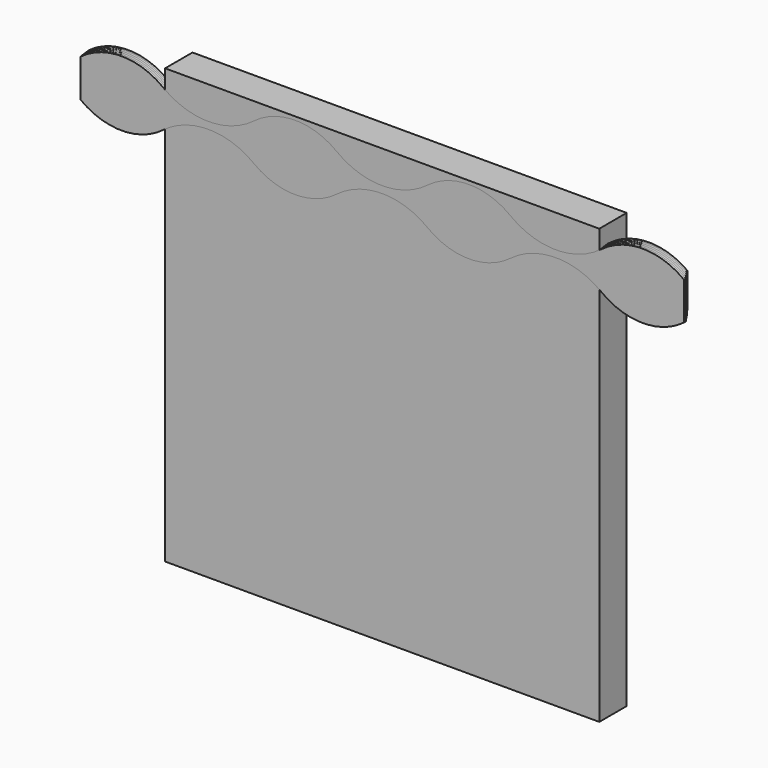
from build123d import *

# Parameters (mm, degrees)
F0_W      = 190
F0_H      = 190
F1_DEPTH  = 15
F3_DEPTH  = 1
F5_DEPTH  = 1
F7_DEPTH  = 1
F9_DEPTH  = 1
F11_DEPTH = 1


with BuildPart() as f1:
    # F0 (on Front) → F1 (new body)
    with BuildSketch(Plane.XZ):
        Rectangle(F0_W, F0_H)
    extrude(amount=-F1_DEPTH)


with BuildPart() as f3:
    # F2 (on face) → F3 (new body)
    with BuildSketch(Plane.XZ):
        with BuildLine():
            ThreePointArc((-56.0905668848, 87.3904664468), (-76, 80.6666666667), (-95.9094331152, 87.3904664468))
            ThreePointArc((-95.9094331152, 87.3904664468), (-114, 93.5), (-132.0905668848, 87.3904664468))
            Line((-132.0905668848, 87.3904664468), (-132.0905668848, 70.9428668865))
            ThreePointArc((-132.0905668848, 70.9428668865), (-114, 64.8333333333), (-95.9094331152, 70.9428668865))
            ThreePointArc((-95.9094331152, 70.9428668865), (-76, 77.6666666667), (-56.0905668848, 70.9428668865))
            ThreePointArc((-56.0905668848, 70.9428668865), (-38, 64.8333333333), (-19.9094331152, 70.9428668865))
            ThreePointArc((-19.9094331152, 70.9428668865), (0, 77.6666666667), (19.9094331152, 70.9428668865))
            ThreePointArc((19.9094331152, 70.9428668865), (38, 64.8333333333), (56.0905668848, 70.9428668865))
            ThreePointArc((56.0905668848, 70.9428668865), (76, 77.6666666667), (95.9094331152, 70.9428668865))
            ThreePointArc((95.9094331152, 70.9428668865), (114, 64.8333333333), (132.0905668848, 70.9428668865))
            Line((132.0905668848, 70.9428668865), (132.0905668848, 87.3904664468))
            ThreePointArc((132.0905668848, 87.3904664468), (114, 93.5), (95.9094331152, 87.3904664468))
            ThreePointArc((95.9094331152, 87.3904664468), (76, 80.6666666667), (56.0905668848, 87.3904664468))
            ThreePointArc((56.0905668848, 87.3904664468), (38, 93.5), (19.9094331152, 87.3904664468))
            ThreePointArc((19.9094331152, 87.3904664468), (0, 80.6666666667), (-19.9094331152, 87.3904664468))
            ThreePointArc((-19.9094331152, 87.3904664468), (-38, 93.5), (-56.0905668848, 87.3904664468))
        make_face()
    extrude(amount=-F3_DEPTH)

    # F4 (on face) → F5 (join)
    with BuildSketch(Plane(origin=(0, 1, 0), x_dir=(-1, 0, 0), z_dir=(0, 1, 0))):
        with BuildLine():
            ThreePointArc((-95.7913197263, 87.4518930814), (-113.6258792589, 93.4999070156), (-131.4905668729, 87.541474107))
            Line((-131.4905668729, 87.541474107), (-131.4905668729, 71.3918592502))
            ThreePointArc((-131.4905668729, 71.3918592502), (-113.6258792589, 65.4334263416), (-95.7913197263, 71.4814402758))
            ThreePointArc((-95.7913197263, 71.4814402758), (-75.6999999881, 78.2666666786), (-55.6086802499, 71.4814402758))
            ThreePointArc((-55.6086802499, 71.4814402758), (-37.6999999881, 65.4333333453), (-19.7913197263, 71.4814402758))
            ThreePointArc((-19.7913197263, 71.4814402758), (0.3000000119, 78.2666666786), (20.3913197501, 71.4814402758))
            ThreePointArc((20.3913197501, 71.4814402758), (38.3000000119, 65.4333333453), (56.2086802737, 71.4814402758))
            ThreePointArc((56.2086802737, 71.4814402758), (76.3000000119, 78.2666666786), (96.3913197501, 71.4814402758))
            ThreePointArc((96.3913197501, 71.4814402758), (114.2258792828, 65.4334263416), (132.0905668967, 71.3918592502))
            Line((132.0905668967, 71.3918592502), (132.0905668967, 87.541474107))
            ThreePointArc((132.0905668967, 87.541474107), (114.2258792828, 93.4999070156), (96.3913197501, 87.4518930814))
            ThreePointArc((96.3913197501, 87.4518930814), (76.3000000119, 80.6666666786), (56.2086802737, 87.4518930814))
            ThreePointArc((56.2086802737, 87.4518930814), (38.3000000119, 93.5000000119), (20.3913197501, 87.4518930814))
            ThreePointArc((20.3913197501, 87.4518930814), (0.3000000119, 80.6666666786), (-19.7913197263, 87.4518930814))
            ThreePointArc((-19.7913197263, 87.4518930814), (-37.6999999881, 93.5000000119), (-55.6086802499, 87.4518930814))
            ThreePointArc((-55.6086802499, 87.4518930814), (-75.6999999881, 80.6666666786), (-95.7913197263, 87.4518930814))
        make_face()
    extrude(amount=F5_DEPTH)

    # F6 (on face) → F7 (join)
    with BuildSketch(Plane(origin=(0, 2, 0), x_dir=(-1, 0, 0), z_dir=(0, 1, 0))):
        with BuildLine():
            ThreePointArc((56.3267936626, 87.513319716), (38.6000000238, 93.5000000238), (20.8732063851, 87.513319716))
            ThreePointArc((20.8732063851, 87.513319716), (0.6000000238, 80.6666666905), (-19.6732063374, 87.513319716))
            ThreePointArc((-19.6732063374, 87.513319716), (-37.3999999762, 93.5000000238), (-55.1267936149, 87.513319716))
            ThreePointArc((-55.1267936149, 87.513319716), (-75.3999999762, 80.6666666905), (-95.6732063374, 87.513319716))
            ThreePointArc((-95.6732063374, 87.513319716), (-113.2520443013, 93.4996256674), (-130.890566861, 87.6915343271))
            Line((-130.890566861, 87.6915343271), (-130.890566861, 71.8417990539))
            ThreePointArc((-130.890566861, 71.8417990539), (-113.2520443013, 66.0337077137), (-95.6732063374, 72.020013665))
            ThreePointArc((-95.6732063374, 72.020013665), (-75.3999999762, 78.8666666905), (-55.1267936149, 72.020013665))
            ThreePointArc((-55.1267936149, 72.020013665), (-37.3999999762, 66.0333333572), (-19.6732063374, 72.020013665))
            ThreePointArc((-19.6732063374, 72.020013665), (0.6000000238, 78.8666666905), (20.8732063851, 72.020013665))
            ThreePointArc((20.8732063851, 72.020013665), (38.6000000238, 66.0333333572), (56.3267936626, 72.020013665))
            ThreePointArc((56.3267936626, 72.020013665), (76.6000000238, 78.8666666905), (96.8732063851, 72.020013665))
            ThreePointArc((96.8732063851, 72.020013665), (114.452044349, 66.0337077137), (132.0905669087, 71.8417990539))
            Line((132.0905669087, 71.8417990539), (132.0905669087, 87.6915343271))
            ThreePointArc((132.0905669087, 87.6915343271), (114.452044349, 93.4996256674), (96.8732063851, 87.513319716))
            ThreePointArc((96.8732063851, 87.513319716), (76.6000000238, 80.6666666905), (56.3267936626, 87.513319716))
        make_face()
    extrude(amount=F7_DEPTH)

    # F8 (on face) → F9 (join)
    with BuildSketch(Plane(origin=(0, 3, 0), x_dir=(-1, 0, 0), z_dir=(0, 1, 0))):
        with BuildLine():
            ThreePointArc((56.4449070515, 87.5747463506), (38.9000000358, 93.5000000358), (21.3550930201, 87.5747463506))
            ThreePointArc((21.3550930201, 87.5747463506), (0.9000000358, 80.6666667024), (-19.5550929485, 87.5747463506))
            ThreePointArc((-19.5550929485, 87.5747463506), (-37.0999999642, 93.5000000358), (-54.6449069799, 87.5747463506))
            ThreePointArc((-54.6449069799, 87.5747463506), (-75.0999999642, 80.6666667024), (-95.5550929485, 87.5747463506))
            ThreePointArc((-95.5550929485, 87.5747463506), (-112.8784991713, 93.49915231), (-130.290566849, 87.8406287996))
            Line((-130.290566849, 87.8406287996), (-130.290566849, 72.2927046052))
            ThreePointArc((-130.290566849, 72.2927046052), (-112.8784991713, 66.6341810948), (-95.5550929485, 72.5585870542))
            ThreePointArc((-95.5550929485, 72.5585870542), (-75.0999999642, 79.4666667024), (-54.6449069799, 72.5585870542))
            ThreePointArc((-54.6449069799, 72.5585870542), (-37.0999999642, 66.6333333691), (-19.5550929485, 72.5585870542))
            ThreePointArc((-19.5550929485, 72.5585870542), (0.9000000358, 79.4666667024), (21.3550930201, 72.5585870542))
            ThreePointArc((21.3550930201, 72.5585870542), (38.9000000358, 66.6333333691), (56.4449070515, 72.5585870542))
            ThreePointArc((56.4449070515, 72.5585870542), (76.9000000358, 79.4666667024), (97.3550930201, 72.5585870542))
            ThreePointArc((97.3550930201, 72.5585870542), (114.6784992428, 66.6341810948), (132.0905669206, 72.2927046052))
            Line((132.0905669206, 72.2927046052), (132.0905669206, 87.8406287996))
            ThreePointArc((132.0905669206, 87.8406287996), (114.6784992428, 93.49915231), (97.3550930201, 87.5747463506))
            ThreePointArc((97.3550930201, 87.5747463506), (76.9000000358, 80.6666667024), (56.4449070515, 87.5747463506))
        make_face()
    extrude(amount=F9_DEPTH)

    # F10 (on face) → F11 (join)
    with BuildSketch(Plane(origin=(0, 4, 0), x_dir=(-1, 0, 0), z_dir=(0, 1, 0))):
        with BuildLine():
            ThreePointArc((-19.4369795597, 87.6361729853), (-36.7999999523, 93.5000000477), (-54.163020345, 87.6361729853))
            ThreePointArc((-54.163020345, 87.6361729853), (-74.7999999523, 80.6666667144), (-95.4369795597, 87.6361729853))
            ThreePointArc((-95.4369795597, 87.6361729853), (-112.5052480041, 93.4984831751), (-129.6905668371, 87.9887386199))
            Line((-129.6905668371, 87.9887386199), (-129.6905668371, 72.7445948088))
            ThreePointArc((-129.6905668371, 72.7445948088), (-112.5052480041, 67.2348502536), (-95.4369795597, 73.0971604434))
            ThreePointArc((-95.4369795597, 73.0971604434), (-74.7999999523, 80.0666667144), (-54.163020345, 73.0971604434))
            ThreePointArc((-54.163020345, 73.0971604434), (-36.7999999523, 67.233333381), (-19.4369795597, 73.0971604434))
            ThreePointArc((-19.4369795597, 73.0971604434), (1.2000000477, 80.0666667144), (21.836979655, 73.0971604434))
            ThreePointArc((21.836979655, 73.0971604434), (39.2000000477, 67.233333381), (56.5630204403, 73.0971604434))
            ThreePointArc((56.5630204403, 73.0971604434), (77.2000000477, 80.0666667144), (97.836979655, 73.0971604434))
            ThreePointArc((97.836979655, 73.0971604434), (114.9052480995, 67.2348502536), (132.0905669325, 72.7445948088))
            Line((132.0905669325, 72.7445948088), (132.0905669325, 87.9887386199))
            ThreePointArc((132.0905669325, 87.9887386199), (114.9052480995, 93.4984831751), (97.836979655, 87.6361729853))
            ThreePointArc((97.836979655, 87.6361729853), (77.2000000477, 80.6666667144), (56.5630204403, 87.6361729853))
            ThreePointArc((56.5630204403, 87.6361729853), (39.2000000477, 93.5000000477), (21.836979655, 87.6361729853))
            ThreePointArc((21.836979655, 87.6361729853), (1.2000000477, 80.6666667144), (-19.4369795597, 87.6361729853))
        make_face()
    extrude(amount=F11_DEPTH)


solid = Compound([f1.part, f3.part])
